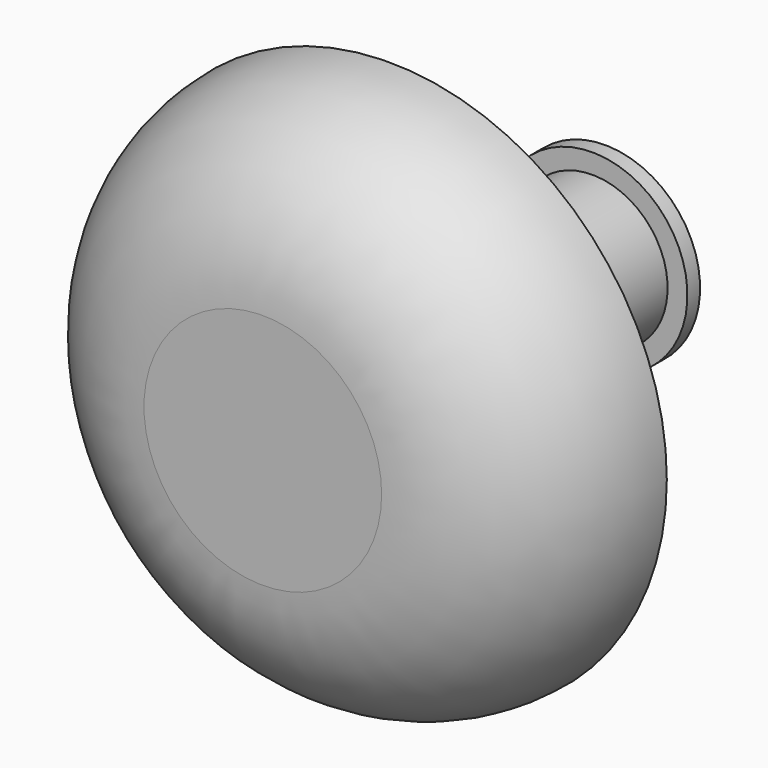
from build123d import *

# Parameters (mm, degrees)
F0_R     = 1.75
F1_DEPTH = 1
F2_R     = 0.99999
F3_R     = 0.475
F4_DEPTH = 1.6
F5_R     = 0.6
F6_DEPTH = 0.1


# Not quite as in the source:
# - a fillet or chamfer is up to 0.001 mm smaller than in the source, because OpenCascade refuses the exact size


with BuildPart() as f1:
    # F0 (on Front) → F1 (new body)
    with BuildSketch(Plane.XZ):
        Circle(F0_R)
    extrude(amount=F1_DEPTH)

    # F2 (radius 1 in the source; OpenCascade refuses exactly that, so slightly less here)
    f2_edges = [f1.edges().sort_by_distance(p)[0] for p in [
        (-1.75, -1, 0),
    ]]
    fillet(f2_edges, radius=F2_R)

    # F3 (on face) → F4 (join)
    with BuildSketch(Plane(origin=(0, 0, 0), x_dir=(-1, 0, 0), z_dir=(0, 1, 0))):
        Circle(F3_R)
    extrude(amount=F4_DEPTH)

    # F5 (on face) → F6 (join)
    with BuildSketch(Plane(origin=(0, 1.6, 0), x_dir=(-1, 0, 0), z_dir=(0, 1, 0))):
        Circle(F5_R)
    extrude(amount=F6_DEPTH)


solid = f1.part
